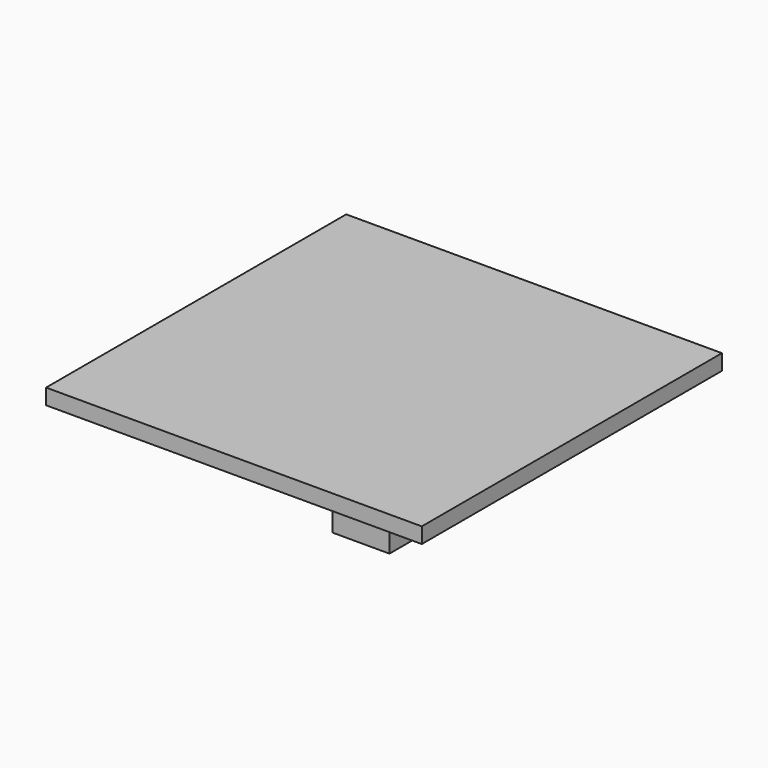
from build123d import *

# Parameters (mm, degrees)
F0_W     = 152.8618186712
F0_H     = 152.6309102774
F1_DEPTH = 6.35
F4_W     = 23.1258999556
F4_H     = 23.3571548015
F5_DEPTH = 50.8


# Not quite as in the source:
# - the program builds the solid bodies; features that only make, move or delete a surface that nothing else refers to are left out


with BuildPart() as f1:
    # F0 (on Top) → F1 (new body)
    with BuildSketch(Plane.XY):
        Rectangle(F0_W, F0_H)
    extrude(amount=F1_DEPTH)

    # F4 (on face) → F5 (join)
    with BuildSketch(Plane(origin=(0, 0, 0), x_dir=(1, 0, 0), z_dir=(0, 0, -1))):
        Rectangle(F4_W, F4_H)
    extrude(amount=F5_DEPTH)


solid = f1.part
